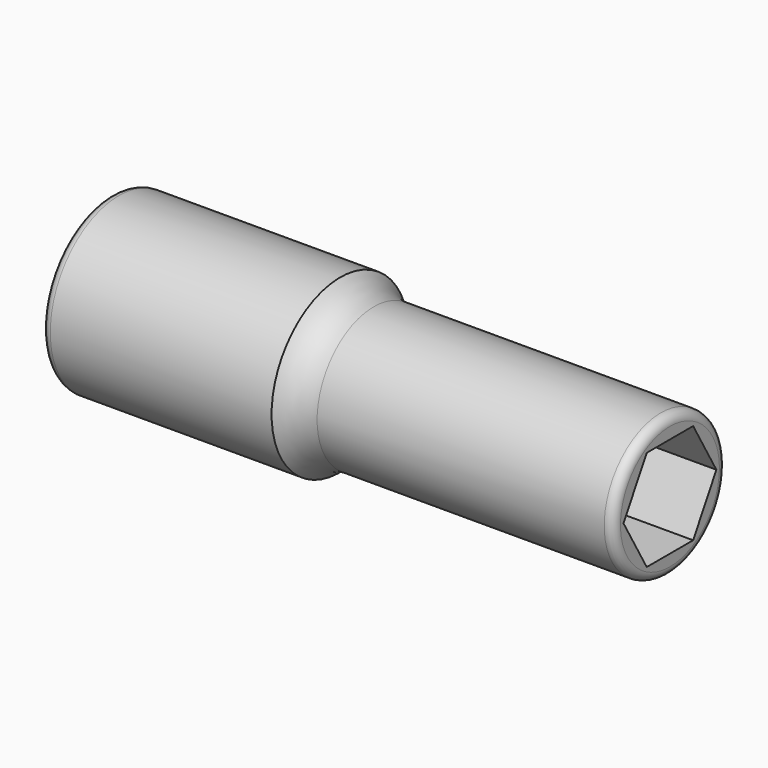
from build123d import *

# Parameters (mm, degrees)
F0_R     = 9.5
F1_DEPTH = 31
F2_R     = 9.5
F2_R_2   = 7.845
F3_DEPTH = 36.5
F5_R     = 1
F7_DEPTH = 29
F8_W     = 9.7
F8_H     = 9.7
F9_DEPTH = 15


# Not quite as in the source:
# - a fillet or chamfer that OpenCascade refuses, or shapes differently, is made with other operations: its cross-section is extruded or revolved along the edge and cut away or added


with BuildPart() as f1:
    # F0 (on Right) → F1 (new body, symmetric)
    with BuildSketch(Plane.YZ):
        Circle(F0_R)
    extrude(amount=F1_DEPTH, both=True)

    # F2 (on face) → F3 (cut)
    with BuildSketch(Plane.YZ.offset(31)):
        Circle(F2_R)
        Circle(F2_R_2, mode=Mode.SUBTRACT)
    extrude(amount=-F3_DEPTH, mode=Mode.SUBTRACT)

    # F4: fillet of radius 5 on 1 edges, made by hand

    # F4_s1 → F4_t2 (revolve)
    with BuildSketch(Plane.XY):
        with BuildLine():
            ThreePointArc((-5.5, 9.5), (-3.8177725447, 8.2774514234), (-1.783687984, 7.845))
            Line((-1.783687984, 7.845), (-5.5, 7.845))
            Line((-5.5, 7.845), (-5.5, 9.5))
        make_face()
    revolve(axis=Axis((-5.5, 0, 0), (1, 0, 0)))

    # F5
    f5_edges = [f1.edges().sort_by_distance(p)[0] for p in [
        (31, -7.845, 0),
        (-31, -9.5, 0),
    ]]
    fillet(f5_edges, radius=F5_R)

    # F6 (on face) → F7 (cut)
    with BuildSketch(Plane.YZ.offset(31)):
        Polygon((3.212954248, 5.565), (-3.212954248, 5.565), (-6.4259084961, 0), (-3.212954248, -5.565), (3.212954248, -5.565), (6.4259084961, 0), align=None)
    extrude(amount=-F7_DEPTH, mode=Mode.SUBTRACT)

    # F8 (on face) → F9 (cut)
    with BuildSketch(Plane(origin=(-31, 0, 0), x_dir=(0, -1, 0), z_dir=(-1, 0, 0))):
        Rectangle(F8_W, F8_H)
    extrude(amount=-F9_DEPTH, mode=Mode.SUBTRACT)


solid = f1.part
